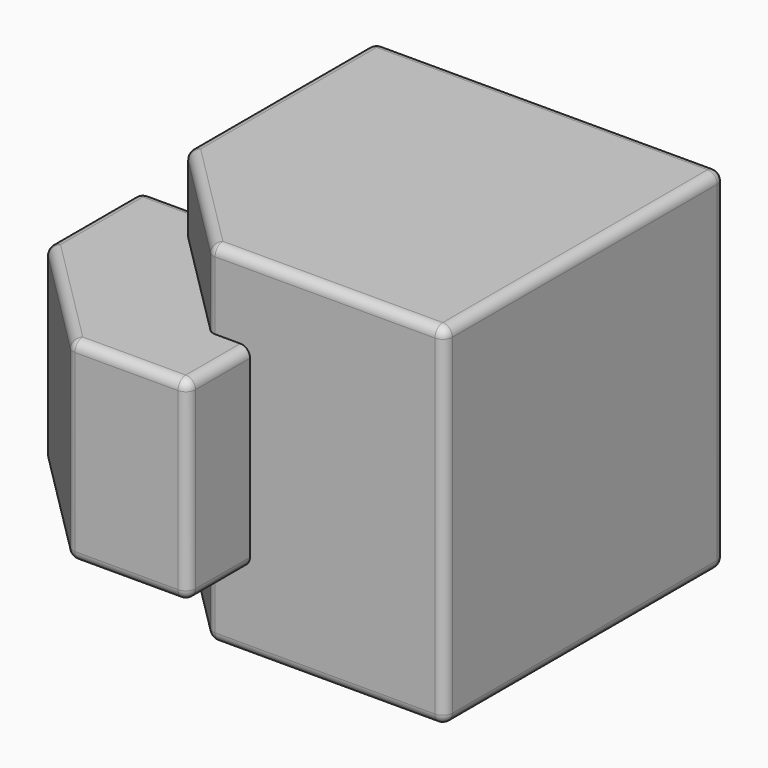
from build123d import *

# Parameters (mm, degrees)
F0_W     = 9
F0_H     = 9
F1_DEPTH = 9
F3_START = 2
F2_W     = 6
F2_H     = 6
F3_DEPTH = 5
F4_SIZE  = 3
F5_SIZE  = 3
F6_SIZE  = 3
F9_R     = 0.25


# Not quite as in the source:
# - a feature of the source that left no trace in its solid (it failed there, or was rolled back) is left out


with BuildPart() as f1:
    # F0 (on Top) → F1 (new body)
    with BuildSketch(Plane.XY):
        Rectangle(F0_W, F0_H)
    extrude(amount=F1_DEPTH)

    # F2 (on Top) → F3 (join)
    with BuildSketch(Plane.XY.offset(F3_START)):
        with Locations((-3.5, -3.5)):
            Rectangle(F2_W, F2_H)
    extrude(amount=F3_DEPTH)

    # F4
    f4_edges = [f1.edges().sort_by_distance(p)[0] for p in [
        (-4.5, -4.5, 1),
    ]]
    chamfer(f4_edges, length=F4_SIZE)

    # F5
    f5_edges = [f1.edges().sort_by_distance(p)[0] for p in [
        (-6.5, -6.5, 4.5),
    ]]
    chamfer(f5_edges, length=F5_SIZE)

    # F6
    f6_edges = [f1.edges().sort_by_distance(p)[0] for p in [
        (-4.5, -4.5, 8),
    ]]
    chamfer(f6_edges, length=F6_SIZE)

    # F9
    f9_edges = [f1.edges().sort_by_distance(p)[0] for p in [
        (-0.5, -6.5, 4.5),
        (-0.5, -5.5, 7),
        (-0.5, -5.5, 2),
        (-2, -6.5, 2),
        (-2, -6.5, 7),
        (-3.5, -6.5, 4.5),
        (-5, -5, 7),
        (-5, -5, 2),
        (-6.5, -3.5, 4.5),
        (-6.5, -2, 7),
        (-6.5, -0.5, 4.5),
        (-6.5, -2, 2),
        (-5.5, -0.5, 2),
        (-5.5, -0.5, 7),
        (-4.5, 1.5, 9),
        (-4.5, -1.5, 8),
        (-4.5, 4.5, 4.5),
        (-4.5, 1.5, 0),
        (-4.5, -1.5, 1),
        (1.5, -4.5, 9),
        (-3, -3, 9),
        (4.5, 0, 9),
        (0, 4.5, 9),
        (-1.5, -4.5, 8),
        (4.5, 4.5, 4.5),
        (0, 4.5, 0),
        (1.5, -4.5, 0),
        (-3, -3, 0),
        (4.5, 0, 0),
        (-1.5, -4.5, 1),
        (4.5, -4.5, 4.5),
    ]]
    fillet(f9_edges, radius=F9_R)


solid = f1.part
